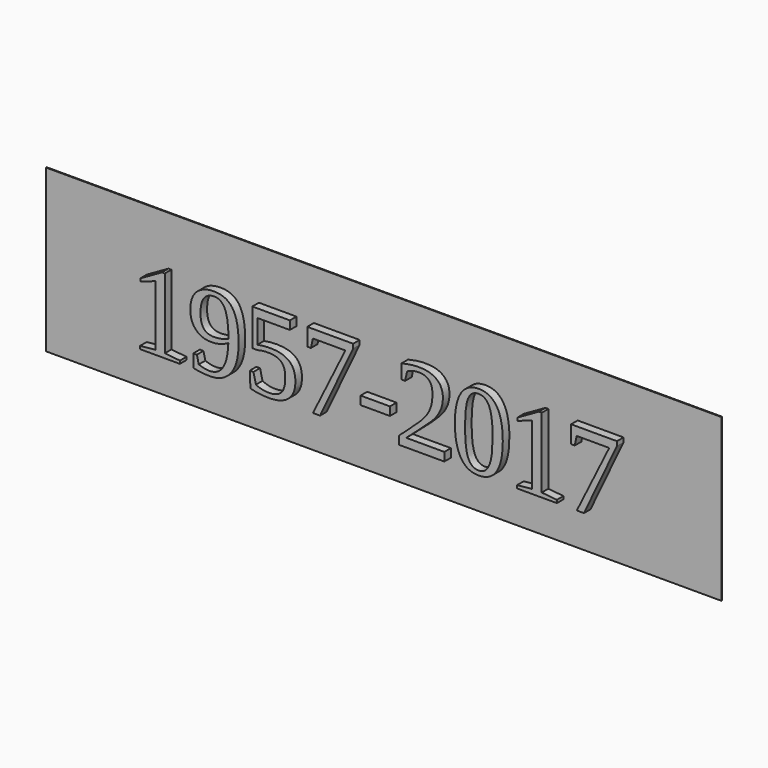
from build123d import *

# Parameters (mm, degrees)
F4_W         = 164.0489697456
F4_H         = 39.3102653325
F5_DEPTH     = 0.2
F6_TEXT_SIZE = 27.4805882563
F7_DEPTH     = 2.2


# Not quite as in the source:
# - Text() gives the source's letters only with a copy of the font that has no kerning and outlines rounded to 1/6400 em; it was checked with that copy


with BuildPart() as f5:
    # F4 (on Front) → F5 (new body)
    with BuildSketch(Plane.XZ):
        Rectangle(F4_W, F4_H)
    extrude(amount=F5_DEPTH)

    # F6 (on Front) → F7 (join)
    with BuildSketch(Plane.XZ):
        with Locations((-60, -10.4224292778)):
            Text('1957-2017', F6_TEXT_SIZE, font='Tinos', text_align=(TextAlign.LEFT, TextAlign.BOTTOM))
    extrude(amount=F7_DEPTH)


solid = f5.part
